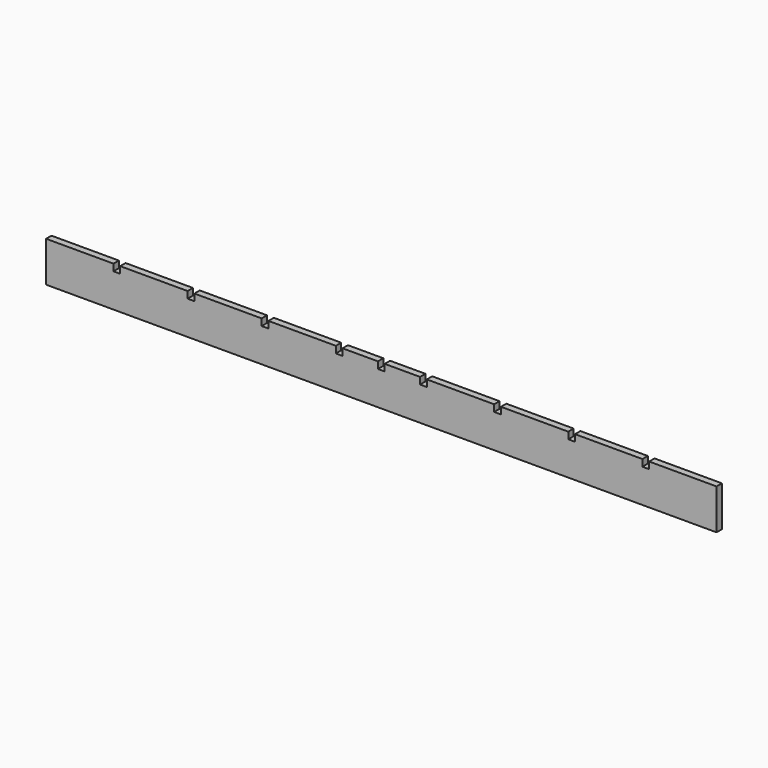
from build123d import *

# Parameters (mm, degrees)
F0_W     = 12.7
F0_H     = 76.2
F1_DEPTH = 1263.65
F2_W     = 12.7
F2_H     = 12.7
F3_DEPTH = 12.7
F5_DEPTH = 12.7


# Not quite as in the source:
# - a feature names something its author has since deleted; it is built from what else it names


with BuildPart() as f1:
    # F0 (on Right) → F1 (new body)
    with BuildSketch(Plane.YZ):
        with Locations((6.35, 38.1)):
            Rectangle(F0_W, F0_H)
    extrude(amount=-F1_DEPTH)

    # F2 (on face) → F3 (cut)
    with BuildSketch(Plane(origin=(0, 12.7, 0), x_dir=(-1, 0, 0), z_dir=(0, 1, 0))):
        with Locations((133.35, 69.85)):
            Rectangle(F2_W, F2_H)
        with Locations((273.05, 69.85)):
            Rectangle(F2_W, F2_H)
        with Locations((412.75, 69.85)):
            Rectangle(F2_W, F2_H)
        with Locations((552.45, 69.85)):
            Rectangle(F2_W, F2_H)
        with Locations((711.2, 69.85)):
            Rectangle(F2_W, F2_H)
        with Locations((850.9, 69.85)):
            Rectangle(F2_W, F2_H)
        with Locations((990.6, 69.85)):
            Rectangle(F2_W, F2_H)
        with Locations((1130.3, 69.85)):
            Rectangle(F2_W, F2_H)
    extrude(amount=-F3_DEPTH, mode=Mode.SUBTRACT)

    # F4 (on face) → F5 (cut)
    with BuildSketch(Plane(origin=(0, 12.7, 0), x_dir=(-1, 0, 0), z_dir=(0, 1, 0))):
        Polygon((631.825, 76.2), (625.475, 76.2), (625.475, 63.5), (638.175, 63.5), (638.175, 76.2), align=None)
    extrude(amount=-F5_DEPTH, mode=Mode.SUBTRACT)


solid = f1.part
